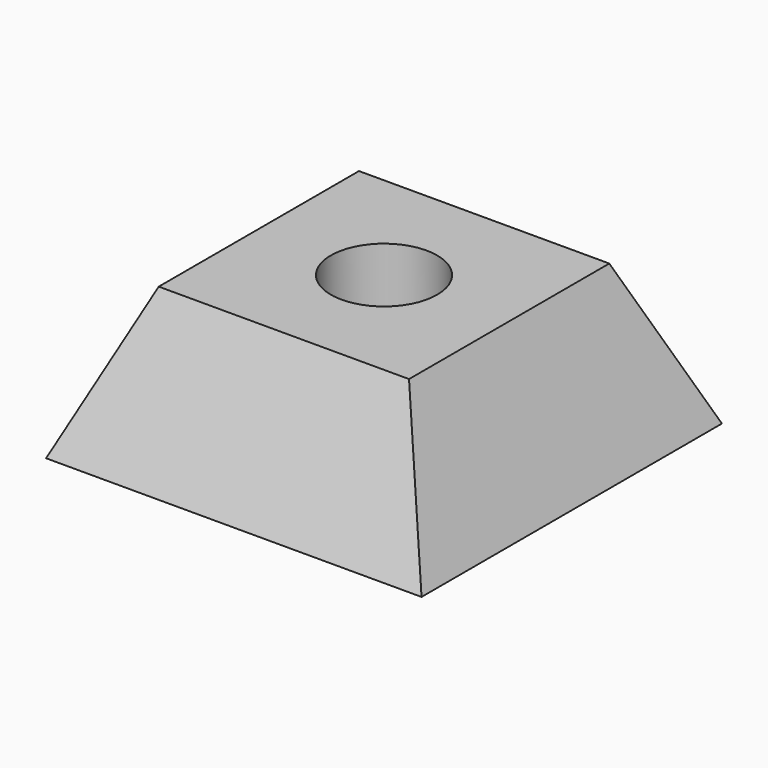
from build123d import *

# Parameters (mm, degrees)
F0_W     = 18
F0_H     = 18
F1_DEPTH = 7
F2_SIZE2 = 6.99999
F2_SIZE  = 2.99999
F3_R     = 2.55
F4_DEPTH = 25


# Not quite as in the source:
# - a fillet or chamfer is up to 0.001 mm smaller than in the source, because OpenCascade refuses the exact size


with BuildPart() as f1:
    # F0 (on Top) → F1 (new body)
    with BuildSketch(Plane.XY):
        Rectangle(F0_W, F0_H)
    extrude(amount=F1_DEPTH)

    # F2 (size 3 and 7 in the source; OpenCascade refuses exactly that, so slightly less here)
    f2_edges = [f1.edges().sort_by_distance(p)[0] for p in [
        (-9, 0, 7),
        (0, 9, 7),
        (9, 0, 7),
        (0, -9, 7),
    ]]
    f2_side = f1.faces().sort_by_distance((0, 0, 7))[0]
    chamfer(f2_edges, length=F2_SIZE, length2=F2_SIZE2, reference=f2_side)

    # F3 (on Top) → F4 (cut)
    with BuildSketch(Plane.XY):
        Circle(F3_R)
    extrude(amount=F4_DEPTH, mode=Mode.SUBTRACT)


solid = f1.part
